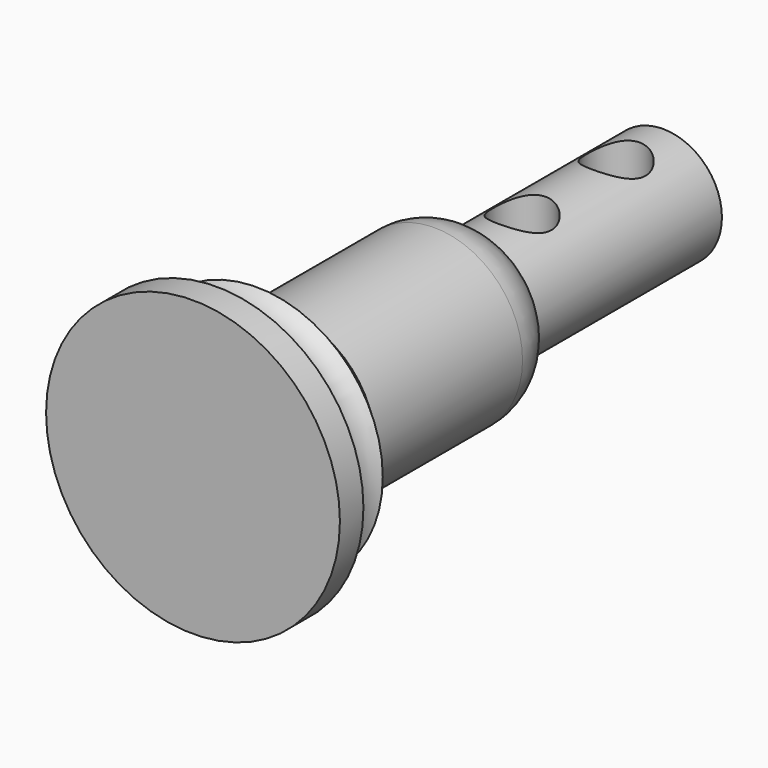
from build123d import *

# Parameters (mm, degrees)
F0_R          = 12.7
F1_DEPTH      = 50.8
F2_R          = 19.05
F3_DEPTH      = 50.8
F4_R          = 31.75
F5_DEPTH      = 25.4
F6_R          = 6.35
F7_DEPTH      = 12.7
F7_DEPTH_BACK = 12.7
F8_R          = 6.35
F9_DEPTH      = 12.7
F9_DEPTH_BACK = 12.7
F13_R         = 6.35
F15_S5_R      = 19.05
F15_T6_DEPTH  = 47


# Not quite as in the source:
# - a fillet or chamfer that OpenCascade refuses, or shapes differently, is made with other operations: its cross-section is extruded or revolved along the edge and cut away or added


with BuildPart() as f1:
    # F0 (on Front) → F1 (new body)
    with BuildSketch(Plane.XZ):
        Circle(F0_R)
    extrude(amount=F1_DEPTH)

    # F2 (on face) → F3 (join)
    with BuildSketch(Plane.XZ.offset(50.8)):
        Circle(F2_R)
    extrude(amount=F3_DEPTH)

    # F4 (on face) → F5 (join)
    with BuildSketch(Plane.XZ.offset(101.6)):
        Circle(F4_R)
    extrude(amount=F5_DEPTH)

    # F6 (on Top) → F7 (cut, two sides)
    with BuildSketch(Plane.XY) as f7_sk:
        with Locations((0, -38.1)):
            Circle(F6_R)
    extrude(amount=-F7_DEPTH, mode=Mode.SUBTRACT)
    extrude(f7_sk.sketch, amount=F7_DEPTH_BACK, mode=Mode.SUBTRACT)

    # F8 (on Top) → F9 (cut, two sides)
    with BuildSketch(Plane.XY) as f9_sk:
        with Locations((0, -12.7)):
            Circle(F8_R)
    extrude(amount=-F9_DEPTH, mode=Mode.SUBTRACT)
    extrude(f9_sk.sketch, amount=F9_DEPTH_BACK, mode=Mode.SUBTRACT)

    # F10: fillet of radius 12.7 on 1 edges, made by hand

    # F10_s1 → F10_t2 (revolve, cut)
    with BuildSketch(Plane.XY):
        with BuildLine():
            ThreePointArc((19.05, -61.7985226281), (17.3485226281, -55.4485226281), (12.7, -50.8))
            Line((12.7, -50.8), (19.05, -50.8))
            Line((19.05, -50.8), (19.05, -61.7985226281))
        make_face()
    revolve(axis=Axis((0, -50.8, 0), (0, -1, 0)), mode=Mode.SUBTRACT)

    # F14: sweep along a path in F12
    with BuildLine(Plane.XZ.offset(114.3)) as f14_path:
        CenterArc((0, 0), 31.75, 0, 360)
    # F13 (on Right) → F14 (sweep, cut)
    with BuildSketch(Plane.YZ):
        with Locations((-114.3, 31.75)):
            Circle(F13_R)
    sweep(path=f14_path.line, mode=Mode.SUBTRACT)

    # F15: chamfer of 12.7 on 1 edges, made by hand


with BuildPart() as f15_tool2:
    # F15_s3 → F15_t4 (revolve)
    with BuildSketch(Plane.XY):
        Polygon((31.75, -114.3), (19.05, -101.6), (31.75, -101.6), align=None)
    revolve(axis=Axis((0, -101.6, 0), (0, -1, 0)))

    # F15_s5 → F15_t6 (cut, symmetric)
    with BuildSketch(Plane.XZ.offset(108)):
        Circle(F15_S5_R)
    extrude(amount=F15_T6_DEPTH, both=True, mode=Mode.SUBTRACT)


with BuildPart() as f1_1:
    add(f1.part)

    # F15_t1: cut F15_tool2
    add(f15_tool2.part, mode=Mode.SUBTRACT)


solid = f1_1.part
